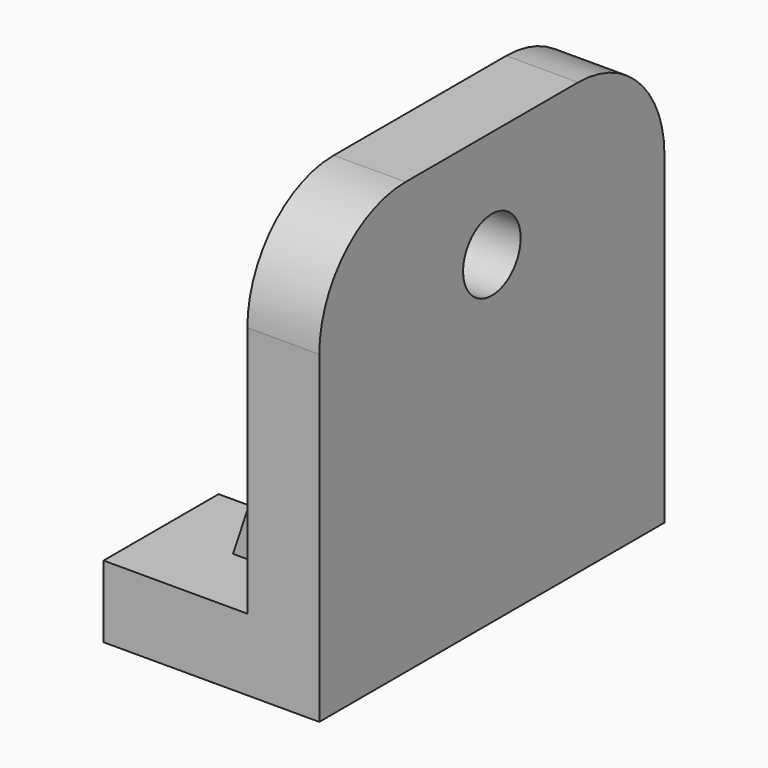
from build123d import *

# Parameters (mm, degrees)
F1_DEPTH = 76.2
F2_R     = 12.7
F3_DEPTH = 76.201
F5_DEPTH = 25.401
F6_R     = 38.1
F9_DEPTH = 6.35


# Not quite as in the source:
# - a pattern or mirror of a feature is missing from the dataset's text; its kind, count and spacing are read off the source's solid


with BuildPart() as f1:
    # F0 (on Front) → F1 (new body, symmetric)
    with BuildSketch(Plane.XZ):
        Polygon((-76.2, 0), (0, 0), (0, 152.4), (-25.4, 152.4), (-25.4, 25.4), (-76.2, 25.4), align=None)
    extrude(amount=F1_DEPTH, both=True)

    # F2 (on Right) → F3 (cut, through all)
    with BuildSketch(Plane.YZ):
        with Locations((0, 114.3)):
            Circle(F2_R)
    extrude(amount=-F3_DEPTH, mode=Mode.SUBTRACT)

    # F4 (on face) → F5 (cut, through all)
    with BuildSketch(Plane.XY.offset(25.4)):
        with BuildLine():
            Line((-63.5, 25.4), (-76.2, 25.4))
            Line((-76.2, 25.4), (-76.2, -25.4))
            Line((-76.2, -25.4), (-63.5, -25.4))
            ThreePointArc((-63.5, -25.4), (-38.1, 0), (-63.5, 25.4))
        make_face()
    extrude(amount=-F5_DEPTH, mode=Mode.SUBTRACT)

    # F6
    f6_edges = [f1.edges().sort_by_distance(p)[0] for p in [
        (-12.7, -76.2, 152.4),
        (-12.7, 76.2, 152.4),
    ]]
    fillet(f6_edges, radius=F6_R)

    # F8 (on offset) → F9 (join, symmetric)
    with BuildSketch(Plane.XZ.offset(44.45)):
        Polygon((-50.8, 25.4), (-25.4, 25.4), (-25.4, 101.6), align=None)
    f9 = extrude(amount=F9_DEPTH, both=True)

    # F9_copies: F9 across plane
    add(f9.mirror(Plane.ZX))


solid = f1.part
